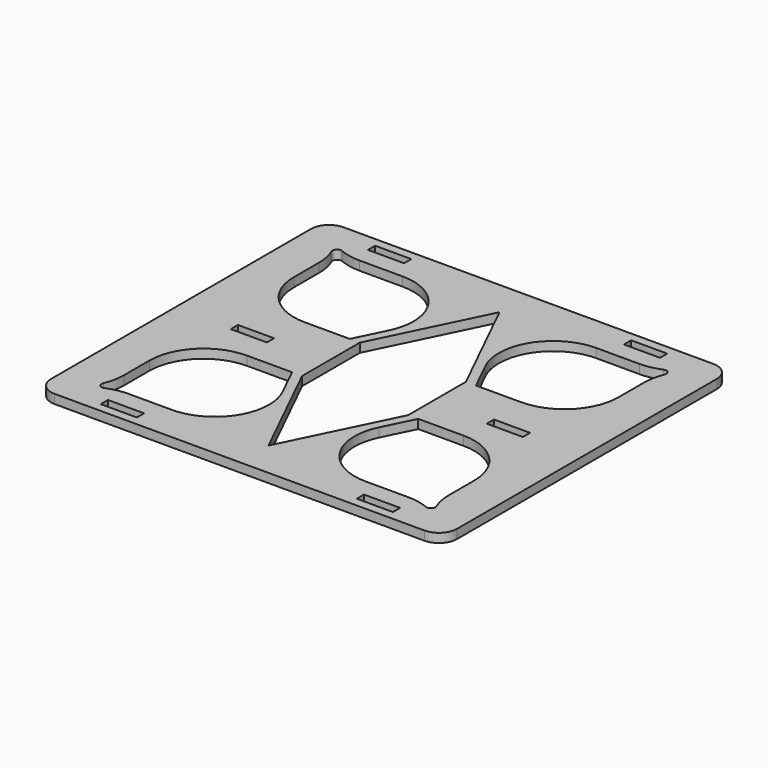
from build123d import *

# Parameters (mm, degrees)
F0_W     = 25.4
F0_H     = 6.35
F1_DEPTH = 6.35
F2_R     = 38.1


# Not quite as in the source:
# - a feature names something its author has since deleted; it is built from what else it names


with BuildPart() as f1:
    # F0 (on Top) → F1 (new body)
    with BuildSketch(Plane.XY):
        with BuildLine():
            ThreePointArc((142.8242, 114.3), (139.1044561211, 123.2802561211), (130.1242, 127))
            Line((130.1242, 127), (-130.1242, 127))
            ThreePointArc((-130.1242, 127), (-139.1044561211, 123.2802561211), (-142.8242, 114.3))
            Line((-142.8242, 114.3), (-142.8242, -114.3))
            ThreePointArc((-142.8242, -114.3), (-139.1044561211, -123.2802561211), (-130.1242, -127))
            Line((-130.1242, -127), (130.1242, -127))
            ThreePointArc((130.1242, -127), (139.1044561211, -123.2802561211), (142.8242, -114.3))
            Line((142.8242, -114.3), (142.8242, 114.3))
        make_face()
        with Locations((-90.0851422843, -117.5192241168)):
            Rectangle(F0_W, F0_H, mode=Mode.SUBTRACT)
        with Locations((-90.0684, -3.175)):
            Rectangle(F0_W, F0_H, mode=Mode.SUBTRACT)
        with Locations((90.0851422843, -117.5192241168)):
            Rectangle(F0_W, F0_H, mode=Mode.SUBTRACT)
        with Locations((90.0684, -3.175)):
            Rectangle(F0_W, F0_H, mode=Mode.SUBTRACT)
        with Locations((-90.0851422843, 117.5192241168)):
            Rectangle(F0_W, F0_H, mode=Mode.SUBTRACT)
        with BuildLine():
            Line((0, 101.6), (7.0708802395, 101.6))
            Line((7.0708802395, 101.6), (111.125, 101.6))
            ThreePointArc((111.125, 101.6), (114.3, 104.775), (117.475, 101.6))
            ThreePointArc((117.475, 101.6), (116.5450640303, 99.3549359697), (114.3, 98.425))
            Line((114.3, 98.425), (114.3, 25.4))
            Line((114.3, 25.4), (44.3961802395, 25.4))
            Line((44.3961802395, 25.4), (37.3253, 25.4))
            Line((37.3253, 25.4), (37.3253, -25.4))
            Line((37.3253, -25.4), (44.3961802395, -25.4))
            Line((44.3961802395, -25.4), (114.3, -25.4))
            Line((114.3, -25.4), (114.3, -98.425))
            ThreePointArc((114.3, -98.425), (116.5450640303, -99.3549359697), (117.475, -101.6))
            ThreePointArc((117.475, -101.6), (114.3, -104.775), (111.125, -101.6))
            Line((111.125, -101.6), (7.0708802395, -101.6))
            Line((7.0708802395, -101.6), (0, -101.6))
            Line((0, -101.6), (-7.0708802395, -101.6))
            Line((-7.0708802395, -101.6), (-111.125, -101.6))
            ThreePointArc((-111.125, -101.6), (-116.5450640303, -103.8450640303), (-114.3, -98.425))
            Line((-114.3, -98.425), (-114.3, -25.4))
            Line((-114.3, -25.4), (-44.3961802395, -25.4))
            Line((-44.3961802395, -25.4), (-37.3253, -25.4))
            Line((-37.3253, -25.4), (-37.3253, 25.4))
            Line((-37.3253, 25.4), (-44.3961802395, 25.4))
            Line((-44.3961802395, 25.4), (-114.3, 25.4))
            Line((-114.3, 25.4), (-114.3, 98.425))
            ThreePointArc((-114.3, 98.425), (-116.5450640303, 103.8450640303), (-111.125, 101.6))
            Line((-111.125, 101.6), (-7.0708802395, 101.6))
            Line((-7.0708802395, 101.6), (0, 101.6))
        make_face(mode=Mode.SUBTRACT)
        with Locations((90.0851422843, 117.5192241168)):
            Rectangle(F0_W, F0_H, mode=Mode.SUBTRACT)
        Polygon((-37.3253, 25.4), (0, 101.6), (-7.0708802395, 101.6), (-44.3961802395, 25.4), align=None)
        Polygon((44.3961802395, 25.4), (7.0708802395, 101.6), (0, 101.6), (37.3253, 25.4), align=None)
        Polygon((44.3961802395, -25.4), (37.3253, -25.4), (0, -101.6), (7.0708802395, -101.6), align=None)
        Polygon((0, -101.6), (-37.3253, -25.4), (-44.3961802395, -25.4), (-7.0708802395, -101.6), align=None)
    extrude(amount=F1_DEPTH)

    # F2
    f2_edges = [f1.edges().sort_by_distance(p)[0] for p in [
        (7.07088, 101.6, 3.175),
        (-7.07088, 101.6, 3.175),
        (114.3, 25.4, 3.175),
        (-114.3, 25.4, 3.175),
        (-114.3, -25.4, 3.175),
        (114.3, -25.4, 3.175),
        (-7.07088, -101.6, 3.175),
        (7.07088, -101.6, 3.175),
        (-114.3, 98.425, 3.175),
        (-111.125, 101.6, 3.175),
        (111.125, 101.6, 3.175),
        (114.3, 98.425, 3.175),
        (114.3, -98.425, 3.175),
        (111.125, -101.6, 3.175),
        (-111.125, -101.6, 3.175),
        (-114.3, -98.425, 3.175),
    ]]
    fillet(f2_edges, radius=F2_R)


solid = f1.part
